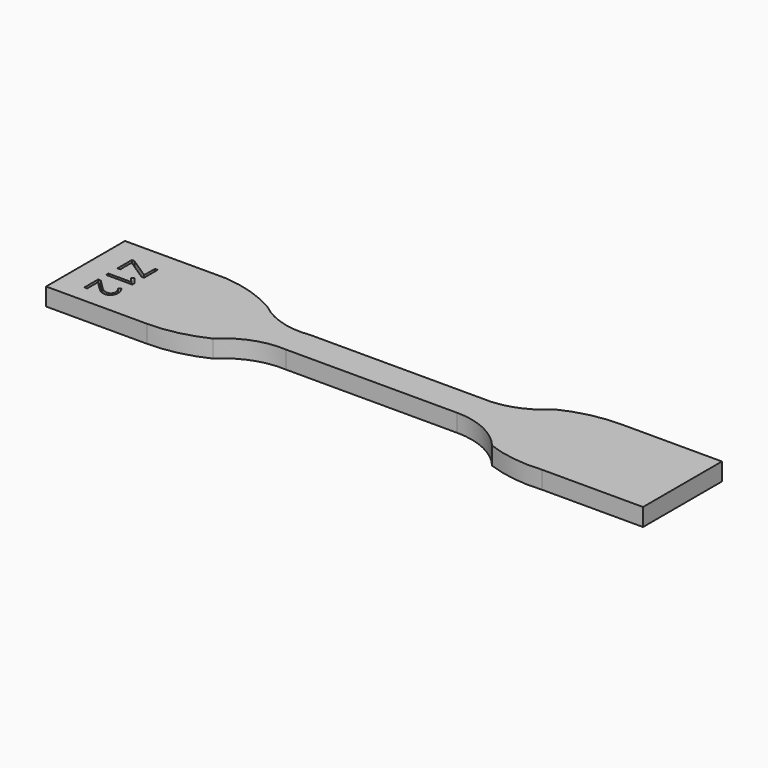
from build123d import *

# Parameters (mm, degrees)
F1_DEPTH     = 3.4
F2_TEXT_SIZE = 7.0564552314
F3_DEPTH     = 1


# Not quite as in the source:
# - Text() gives the source's letters only with a copy of the font that has no kerning and outlines rounded to 1/6400 em; it was checked with that copy


with BuildPart() as f1:
    # F0 (on Top) → F1 (new body)
    with BuildSketch(Plane.XY):
        with BuildLine():
            Line((-14.4320548165, 19.7811394548), (-33.8720548165, 19.7811394548))
            Line((-33.8720548165, 19.7811394548), (-33.8720548165, 0.7811394548))
            Line((-33.8720548165, 0.7811394548), (-14.4320548165, 0.7811394548))
            ThreePointArc((-14.4320548165, 0.7811394548), (-8.9053122052, 1.3996892086), (-3.6520548165, 3.2247301661))
            ThreePointArc((-3.6520548165, 3.2247301661), (1.3014698263, 6.4128780055), (7.1279451835, 7.2811394548))
            Line((7.1279451835, 7.2811394548), (40.1279451835, 7.2811394548))
            ThreePointArc((40.1279451835, 7.2811394548), (46.0837574042, 5.9511158081), (50.9079451835, 2.2137538538))
            ThreePointArc((50.9079451835, 2.2137538538), (56.2191047011, 0.9041953221), (61.6879451835, 0.7811394548))
            Line((61.6879451835, 0.7811394548), (81.1279451835, 0.7811394548))
            Line((81.1279451835, 0.7811394548), (81.1279451835, 19.7811394548))
            Line((81.1279451835, 19.7811394548), (61.6879451835, 19.7811394548))
            ThreePointArc((61.6879451835, 19.7811394548), (56.1612025723, 19.162589701), (50.9079451835, 17.3375487435))
            ThreePointArc((50.9079451835, 17.3375487435), (45.9544205407, 14.1494009041), (40.1279451835, 13.2811394548))
            Line((40.1279451835, 13.2811394548), (7.1279451835, 13.2811394548))
            ThreePointArc((7.1279451835, 13.2811394548), (1.4167452884, 13.6925537245), (-3.6520548165, 16.3560723447))
            ThreePointArc((-3.6520548165, 16.3560723447), (-8.8458057958, 18.686276846), (-14.4320548165, 19.7811394548))
        make_face()
    extrude(amount=F1_DEPTH)

    # F2 (on face) → F3 (cut)
    with BuildSketch(Plane.XY.offset(3.4)):
        with Locations(Location((-29.1824135929, 15.8650862949), (0, 0, -90))):
            Text('Z12', F2_TEXT_SIZE, font='Open Sans', text_align=(TextAlign.LEFT, TextAlign.BOTTOM))
    extrude(amount=-F3_DEPTH, mode=Mode.SUBTRACT)


solid = f1.part
